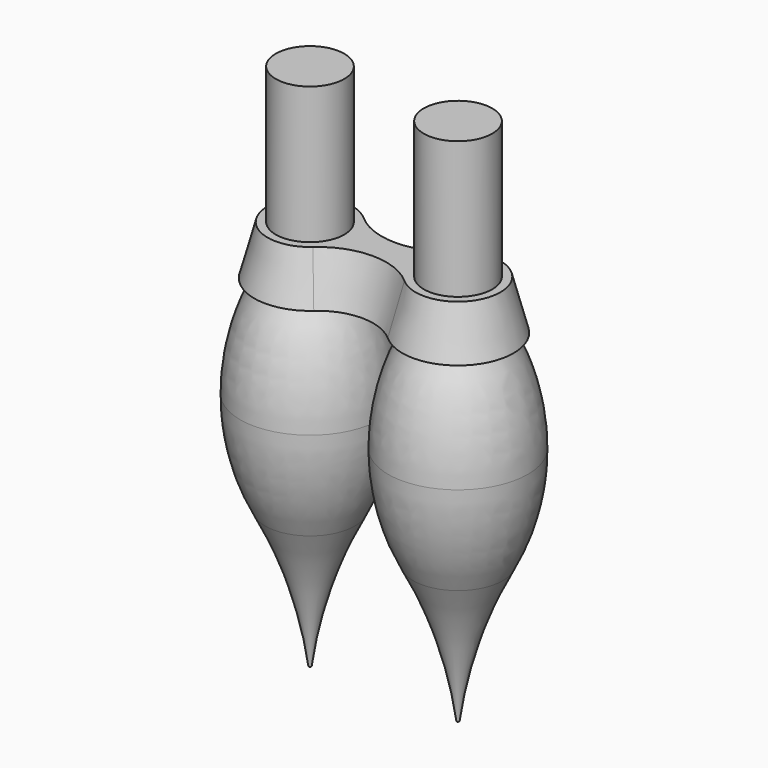
from build123d import *

# Parameters (mm, degrees)
F4_DEPTH = 4.572
F4_TAPER = 15


with BuildPart() as f1:
    # F0 (on Front) → F1 (revolve)
    with BuildSketch(Plane.XZ):
        with BuildLine():
            Line((-6.858, 12.7), (-10.033, 12.7))
            Line((-10.033, 12.7), (-10.033, -4.572))
            Line((-10.033, -4.572), (-10.9982, -4.572))
            ThreePointArc((-10.9982, -4.572), (-12.7421516444, -9.1602447444), (-13.335, -14.0328095721))
            ThreePointArc((-13.335, -14.0328095721), (-12.7463257854, -18.8884436966), (-11.0144111466, -23.4627405568))
            ThreePointArc((-11.0144111466, -23.4627405568), (-8.4355524205, -29.6589038682), (-6.9839312526, -36.2114413992))
            ThreePointArc((-6.9839312526, -36.2114413992), (-6.9417882519, -36.290438613), (-6.858, -36.322))
            Line((-6.858, -36.322), (-6.858, 12.7))
        make_face()
    revolve(axis=Axis((-6.858, 0, -6.3344838709), (0, 0, -1)))


with BuildPart() as f2_1:
    # F2: instance of F1
    add(f1.part.mirror(Plane.YZ))


with BuildPart() as f1_1:
    add(f1.part)

    add(f2_1.part)  # F4 merges F2_1
    # F3 (on face) → F4 (join)
    with BuildSketch(Plane.XY.offset(-4.572)):
        with BuildLine():
            ThreePointArc((3.429, 3.8507606314), (0, 2.5453212627), (-3.429, 3.8507606314))
            ThreePointArc((-3.429, 3.8507606314), (-12.0142, 0), (-3.429, -3.8507606314))
            ThreePointArc((-3.429, -3.8507606314), (0, -2.5453212627), (3.429, -3.8507606314))
            ThreePointArc((3.429, -3.8507606314), (12.0142, 0), (3.429, 3.8507606314))
        make_face()
    extrude(amount=F4_DEPTH, taper=F4_TAPER)


solid = f1_1.part
